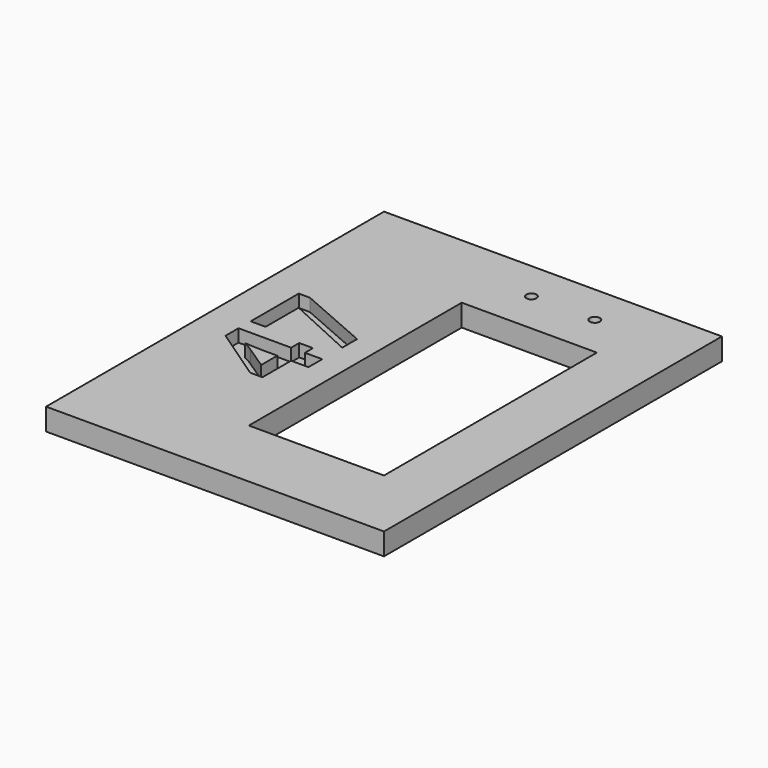
from build123d import *

# Parameters (mm, degrees)
F0_W         = 40
F0_H         = 50
F1_DEPTH     = 2.6
F2_TEXT_SIZE = 13.8888888889
F3_DEPTH     = 1.5
F4_W         = 16
F4_H         = 31.5
F4_R         = 0.6
F5_DEPTH     = 2.6


# Not quite as in the source:
# - Text() gives the source's letters only with a copy of the font that has no kerning and outlines rounded to 1/6400 em; it was checked with that copy


with BuildPart() as f1:
    # F0 (on Top) → F1 (new body)
    with BuildSketch(Plane.XY):
        with Locations((-23.1587231159, 3.3350909071)):
            Rectangle(F0_W, F0_H)
    extrude(amount=F1_DEPTH)

    # F2 (on face) → F3 (cut)
    with BuildSketch(Plane.XY.offset(2.6)):
        with Locations(Location((-29.1587231159, -4.8149090929), (0, 0, 90))):
            Text('47', F2_TEXT_SIZE, font='Open Sans', font_style=FontStyle.BOLD, text_align=(TextAlign.LEFT, TextAlign.BOTTOM))
    extrude(amount=-F3_DEPTH, mode=Mode.SUBTRACT)

    # F4 (on face) → F5 (cut, through all)
    with BuildSketch(Plane.XY.offset(2.6)):
        with Locations((-18.1587231159, 2.8350909071)):
            Rectangle(F4_W, F4_H)
        with Locations((-21.9087231159, 23.5850909071)):
            Circle(F4_R)
        with Locations((-14.4087231159, 23.5850909071)):
            Circle(F4_R)
    extrude(amount=-F5_DEPTH, mode=Mode.SUBTRACT)


solid = f1.part
